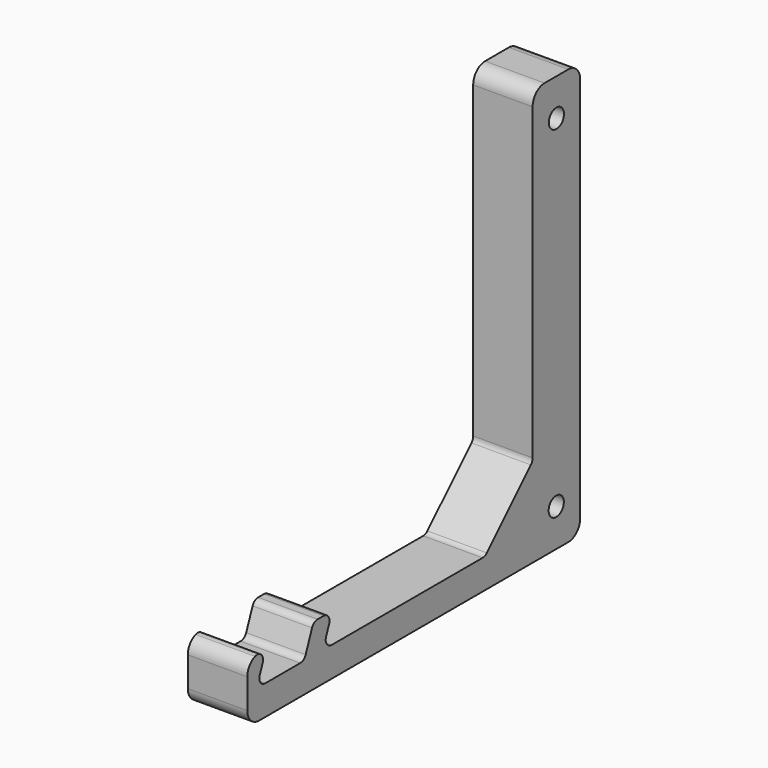
from build123d import *

# Parameters (mm, degrees)
F1_DEPTH = 25.4
F2_SIZE  = 25.4
F3_R     = 6.35
F4_R     = 3.175
F5_R     = 4.05
F6_DEPTH = 25.4010001


with BuildPart() as f1:
    # F0 (on Right) → F1 (new body)
    with BuildSketch(Plane.YZ):
        Polygon((-177.8, 0), (0, 0), (0, 177.8), (-25.3918121044, 177.8), (-25.3918121044, 12.7), (-137.4, 12.7), (-132.4, 25.4), (-142.4, 25.4), (-147.4, 12.7), (-172.8, 12.7), (-167.8, 25.4), (-177.8, 25.4), align=None)
    extrude(amount=F1_DEPTH)

    # F2
    f2_edges = [f1.edges().sort_by_distance(p)[0] for p in [
        (12.7, -25.391812, 12.7),
    ]]
    chamfer(f2_edges, length=F2_SIZE)

    # F3
    f3_edges = [f1.edges().sort_by_distance(p)[0] for p in [
        (12.7, 0, 0),
        (12.7, 0, 177.8),
        (12.7, -25.391812, 177.8),
        (12.7, -177.8, 25.4),
        (12.7, -177.8, 0),
    ]]
    fillet(f3_edges, radius=F3_R)

    # F4
    f4_edges = [f1.edges().sort_by_distance(p)[0] for p in [
        (12.7, -172.8, 12.7),
        (12.7, -137.4, 12.7),
        (12.7, -147.4, 12.7),
        (12.7, -142.4, 25.4),
        (12.7, -132.4, 25.4),
        (12.7, -167.8, 25.4),
        (12.7, -25.391812, 38.1),
        (12.7, -50.791812, 12.7),
    ]]
    fillet(f4_edges, radius=F4_R)

    # F5 (on face) → F6 (cut, through all)
    with BuildSketch(Plane.YZ.offset(25.4)):
        with Locations((-12.7061052421, 161.9854427668)):
            Circle(F5_R)
        with Locations((-12.8001880162, 16.1035214467)):
            Circle(F5_R)
    extrude(amount=-F6_DEPTH, mode=Mode.SUBTRACT)


solid = f1.part
